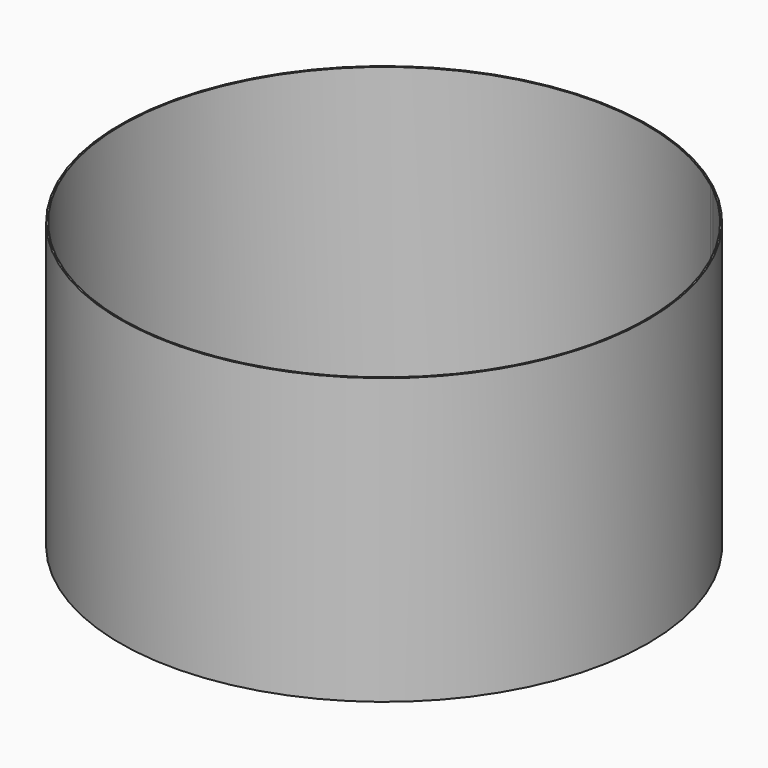
from build123d import *

# Parameters (mm, degrees)
F1_DEPTH = 25
F0_R     = 265
F0_R_2   = 880
F2_DEPTH = 950


with BuildPart() as f1:
    # F0 (on Top) → F1 (new body)
    with BuildSketch(Plane.XY):
        with BuildLine():
            ThreePointArc((-193.9061843773, -853.2440399207), (30.141564439, -801.9408802065), (129.8196926395, -594.8329887472))
            ThreePointArc((129.8196926395, -594.8329887472), (128.8042074457, -571.6559323656), (125.7655345828, -548.6565058525))
            ThreePointArc((125.7655345828, -548.6565058525), (122.470052193, -535.7732038744), (119.8250195137, -522.7408028614))
            ThreePointArc((119.8250195137, -522.7408028614), (-76.4544361301, -336.4219362587), (-333.9813542907, -419.6098631631))
            ThreePointArc((-333.9813542907, -419.6098631631), (-341.9991199047, -430.2190624071), (-350.5390087439, -440.4126865248))
            ThreePointArc((-350.5390087439, -440.4126865248), (-382.9463676187, -688.8381980929), (-193.9061843773, -853.2440399207))
        make_face()
    extrude(amount=F1_DEPTH)


with BuildPart() as f1b:
    # F0 (on Top) → F1, piece 2 (new body)
    with BuildSketch(Plane.XY):
        with BuildLine():
            ThreePointArc((119.8250195137, -522.7408028614), (123.1205019034, -535.6241048395), (125.7655345828, -548.6565058525))
            ThreePointArc((125.7655345828, -548.6565058525), (299.7849702857, -728.8861094166), (546.1877145957, -683.5963578199))
            ThreePointArc((546.1877145957, -683.5963578199), (619.5808969263, -591.4327967526), (645.7708614569, -476.5643199667))
            ThreePointArc((645.7708614569, -476.5643199667), (609.6849391517, -343.0602187819), (511.2550498858, -245.9155034294))
            ThreePointArc((511.2550498858, -245.9155034294), (495.1315212016, -238.8100345014), (479.5158115711, -230.6488165373))
            ThreePointArc((479.5158115711, -230.6488165373), (213.7178326121, -270.8502330554), (119.8250195137, -522.7408028614))
        make_face()
    extrude(amount=F1_DEPTH)


with BuildPart() as f1c:
    # F0 (on Top) → F1, piece 3 (new body)
    with BuildSketch(Plane.XY):
        with BuildLine():
            ThreePointArc((-787.9877787267, -380.3948745413), (-585.3605198344, -527.7300838352), (-350.5390087439, -440.4126865248))
            ThreePointArc((-350.5390087439, -440.4126865248), (-342.52124313, -429.8034872808), (-333.9813542907, -419.6098631631))
            ThreePointArc((-333.9813542907, -419.6098631631), (-297.0554387565, -346.2911766256), (-284.3400556741, -265.1895609407))
            ThreePointArc((-284.3400556741, -265.1895609407), (-357.4011316606, -82.4754414848), (-536.2981647198, -0.5106817676))
            ThreePointArc((-536.2981647198, -0.5106817676), (-549.5917623332, -0.8570003073), (-562.8859953912, -0.5359996249))
            ThreePointArc((-562.8859953912, -0.5359996249), (-777.3172521182, -130.0918263132), (-787.9877787267, -380.3948745413))
        make_face()
    extrude(amount=F1_DEPTH)


with BuildPart() as f1d:
    # F0 (on Top) → F1, piece 4 (new body)
    with BuildSketch(Plane.XY):
        with BuildLine():
            ThreePointArc((495.0207504098, 238.7567217141), (345.1444456193, 8.7484463585), (479.5158115711, -230.6488165373))
            ThreePointArc((479.5158115711, -230.6488165373), (495.6393402554, -237.7542854654), (511.2550498858, -245.9155034294))
            ThreePointArc((511.2550498858, -245.9155034294), (758.421002927, -219.5363429825), (875, 0))
            ThreePointArc((875, 0), (750.9884726823, 224.3819301341), (495.0207504098, 238.7567217141))
        make_face()
    extrude(amount=F1_DEPTH)


with BuildPart() as f1e:
    # F0 (on Top) → F1, piece 5 (new body)
    with BuildSketch(Plane.XY):
        with BuildLine():
            ThreePointArc((-788.7107999512, 378.8934864053), (-777.5635978963, 128.6112142499), (-562.8859953912, -0.5359996249))
            ThreePointArc((-562.8859953912, -0.5359996249), (-549.5923977778, -0.1896810852), (-536.2981647198, -0.5106817676))
            ThreePointArc((-536.2981647198, -0.5106817676), (-357.7312807823, 81.6116137676), (-284.8441044368, 264.1428795483))
            ThreePointArc((-284.8441044368, 264.1428795483), (-297.6368296433, 345.4846925427), (-334.7798821065, 418.9730454509))
            ThreePointArc((-334.7798821065, 418.9730454509), (-343.339168888, 429.1503871388), (-351.3771248405, 439.7442975662))
            ThreePointArc((-351.3771248405, 439.7442975662), (-586.3645037542, 526.6143264405), (-788.7107999512, 378.8934864053))
        make_face()
    extrude(amount=F1_DEPTH)


with BuildPart() as f1f:
    # F0 (on Top) → F1, piece 6 (new body)
    with BuildSketch(Plane.XY):
        with BuildLine():
            ThreePointArc((119.2137956135, 524.3526253699), (219.7006191662, 266.525760103), (495.0207504098, 238.7567217141))
            ThreePointArc((495.0207504098, 238.7567217141), (604.4234298179, 336.5249707271), (645.0414992079, 477.5134426521))
            ThreePointArc((645.0414992079, 477.5134426521), (621.8583685619, 585.9090223399), (556.365259994, 675.3389500627))
            ThreePointArc((556.365259994, 675.3389500627), (544.884833308, 684.6353178379), (533.2491005483, 693.7365470872))
            ThreePointArc((533.2491005483, 693.7365470872), (290.8989625906, 727.0702661722), (124.5148010842, 547.7352807511))
            ThreePointArc((124.5148010842, 547.7352807511), (122.1288785288, 535.9839709516), (119.2137956135, 524.3526253699))
        make_face()
    extrude(amount=F1_DEPTH)


with BuildPart() as f1g:
    # F0 (on Top) → F1, piece 7 (new body)
    with BuildSketch(Plane.XY):
        with BuildLine():
            ThreePointArc((-195.5307848239, 852.8732099123), (-384.2575390444, 688.1076512362), (-351.3771248405, 439.7442975662))
            ThreePointArc((-351.3771248405, 439.7442975662), (-342.817838059, 429.5669558783), (-334.7798821065, 418.9730454509))
            ThreePointArc((-334.7798821065, 418.9730454509), (-76.3949015791, 336.4372263944), (119.2137956135, 524.3526253699))
            ThreePointArc((119.2137956135, 524.3526253699), (121.599718169, 536.1039351694), (124.5148010842, 547.7352807511))
            ThreePointArc((124.5148010842, 547.7352807511), (127.6419624313, 571.062141726), (128.6870974898, 594.5744634688))
            ThreePointArc((128.6870974898, 594.5744634688), (28.8116886125, 801.8396786077), (-195.5307848239, 852.8732099123))
        make_face()
    extrude(amount=F1_DEPTH)


with BuildPart() as f1h:
    # F0 (on Top) → F1, piece 8 (new body)
    with BuildSketch(Plane.XY):
        Circle(F0_R)
    extrude(amount=F1_DEPTH)


with BuildPart() as f2:
    # F0 (on Top) → F2 (new body)
    with BuildSketch(Plane.XY):
        Circle(F0_R_2)
        with BuildLine():
            ThreePointArc((546.1877145957, -683.5963578199), (195.5010310556, -852.8800307524), (-193.9061843773, -853.2440399207))
            ThreePointArc((-193.9061843773, -853.2440399207), (-544.9087281325, -684.6162998388), (-787.9877787267, -380.3948745413))
            ThreePointArc((-787.9877787267, -380.3948745413), (-874.9996032962, -0.8332055607), (-788.7107999512, 378.8934864053))
            ThreePointArc((-788.7107999512, 378.8934864053), (-546.211560546, 683.5773044257), (-195.5307848239, 852.8732099123))
            ThreePointArc((-195.5307848239, 852.8732099123), (186.6669080413, 854.8569853738), (533.2491005483, 693.7365470872))
            ThreePointArc((533.2491005483, 693.7365470872), (545.0637630098, 684.8601389116), (556.365259994, 675.3389500627))
            ThreePointArc((556.365259994, 675.3389500627), (791.3420886364, 373.3667081471), (875, 0))
            ThreePointArc((875, 0), (788.5236997932, -379.2827110011), (546.1877145957, -683.5963578199))
        make_face(mode=Mode.SUBTRACT)
    extrude(amount=F2_DEPTH)


solid = Compound([f1.part, f1b.part, f1c.part, f1d.part, f1e.part, f1f.part, f1g.part, f1h.part, f2.part])
